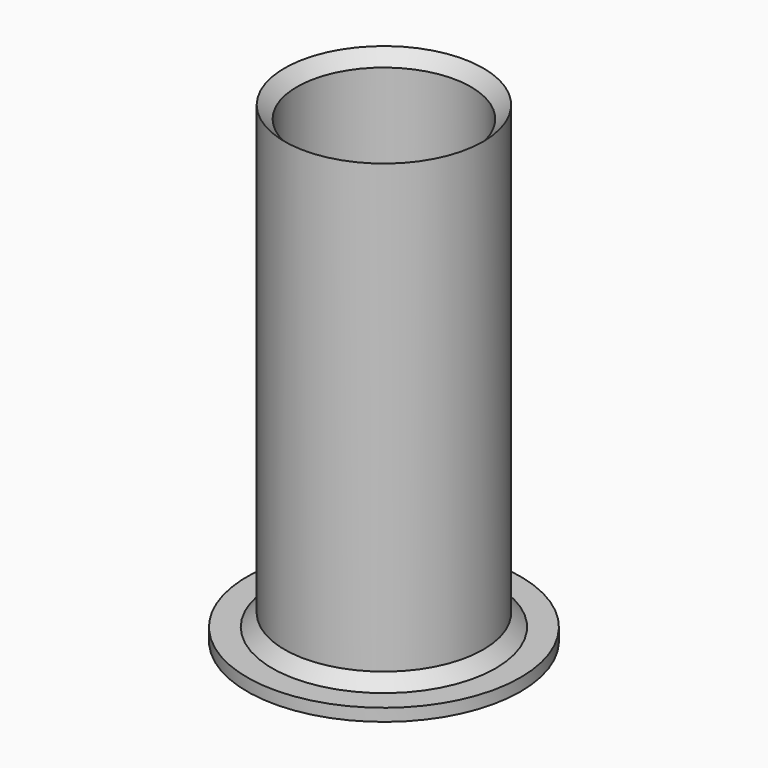
from build123d import *

# Parameters (mm, degrees)
F0_R     = 11
F0_R_2   = 8
F1_DEPTH = 1
F0_R_3   = 7
F2_DEPTH = 39
F3_SIZE  = 1


# Not quite as in the source:
# - a fillet or chamfer that OpenCascade refuses, or shapes differently, is made with other operations: its cross-section is extruded or revolved along the edge and cut away or added


with BuildPart() as f1:
    # F0 (on Top) → F1 (new body)
    with BuildSketch(Plane.XY):
        Circle(F0_R)
        Circle(F0_R_2, mode=Mode.SUBTRACT)
    extrude(amount=F1_DEPTH)

    # F0 (on Top) → F2 (join)
    with BuildSketch(Plane.XY):
        Circle(F0_R_2)
        Circle(F0_R_3, mode=Mode.SUBTRACT)
    extrude(amount=F2_DEPTH)

    # F3
    f3_edges = [f1.edges().sort_by_distance(p)[0] for p in [
        (-8, 0, 1),
        (-7, 0, 0),
    ]]
    chamfer(f3_edges, length=F3_SIZE)

    # F4: chamfer of 2 on 1 edges, made by hand

    # F4_s1 → F4_t2 (revolve, cut)
    with BuildSketch(Plane.XZ):
        Polygon((7, 37), (9, 39), (7, 39), align=None)
    revolve(axis=Axis((0, 0, 39), (0, 0, 1)), mode=Mode.SUBTRACT)


solid = f1.part
